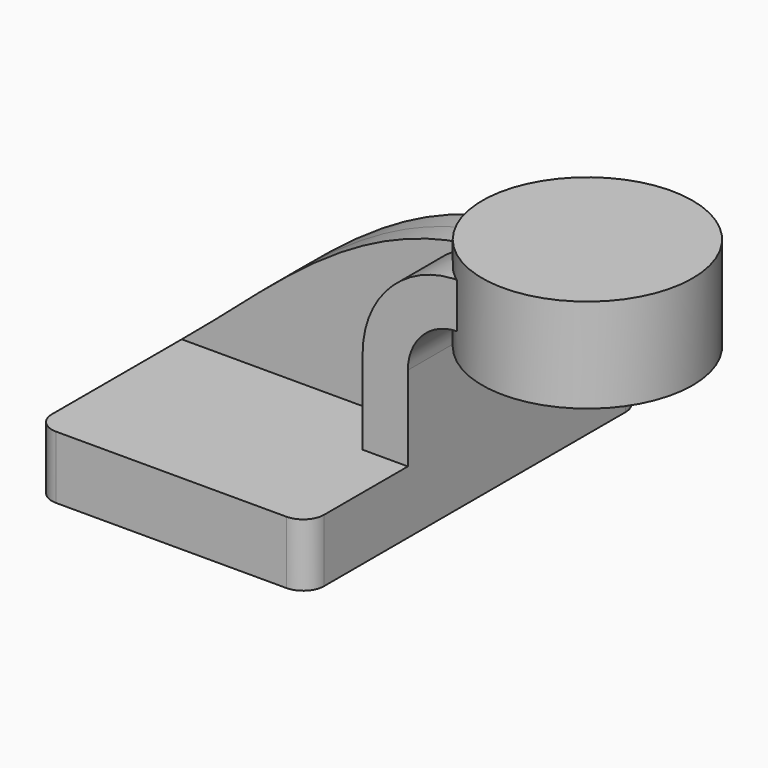
from build123d import *

# Parameters (mm, degrees)
F1_DEPTH = 63.5
F2_DEPTH = 7.9375
F3_DEPTH = 25.4
F4_R     = 6.35


# Not quite as in the source:
# - ends of sketch curves that miss each other by under 0.0002 mm in the source are joined


with BuildPart() as f1:
    # F0 (on Front) → F1 (new body, symmetric)
    with BuildSketch(Plane.XZ):
        Polygon((-41.275, 9.525), (-41.275, -9.525), (41.275, -9.525), (41.275, 9.525), (27.5589991361, 9.525), align=None)
    extrude(amount=F1_DEPTH, both=True)

    # F0 (on Front) → F2 (join, symmetric)
    with BuildSketch(Plane.XZ):
        with BuildLine():
            add(Edge.make_bspline(
                [(-41.275, 9.525), (-12.8610799571, 32.6827113613), (12.6950968294, 62.5117734864), (54.8244975817, 64.1265564996)],
                knots=[0, 0, 0, 0, 110.5540678871, 110.5540678871, 110.5540678871, 110.5540678871], degree=3))
            Line((-41.275, 9.525), (27.5589991361, 9.525))
            Line((27.5589991361, 9.525), (27.5589991361, 35.2199450135))
            ThreePointArc((27.5589991361, 35.2199450135), (35.450810299, 55.0882589398), (54.8244975817, 64.1265564996))
        make_face()
    extrude(amount=F2_DEPTH, both=True)

    # F0 (on Front) → F3 (join, symmetric)
    with BuildSketch(Plane.XZ):
        with BuildLine():
            Line((27.5589991361, 9.525), (41.275, 9.525))
            Line((41.275, 9.525), (41.275, 35.2199450135))
            ThreePointArc((41.275, 35.2199450135), (45.7386926547, 45.9962523588), (56.515, 50.4599450135))
            Line((56.515, 50.4599450135), (56.515, 64.1759467518))
            add(Edge.make_bspline(
                [(54.8244975817, 64.1265564996), (55.3850490812, 64.1480419473), (55.9485346305, 64.1645324648), (56.515, 64.1759467518)],
                knots=[110.5540678871, 110.5540678871, 110.5540678871, 110.5540678871, 112.0250417777, 112.0250417777, 112.0250417777, 112.0250417777], degree=3))
            ThreePointArc((54.8244975817, 64.1265564996), (35.450810299, 55.0882589398), (27.5589991361, 35.2199450135))
            Line((27.5589991361, 35.2199450135), (27.5589991361, 9.525))
        make_face()
    extrude(amount=F3_DEPTH, both=True)

    # F4
    f4_edges = [f1.edges().sort_by_distance(p)[0] for p in [
        (-41.275, -63.5, 0),
        (41.275, -63.5, 0),
        (41.275, 63.5, 0),
        (-41.275, 63.5, 0),
    ]]
    fillet(f4_edges, radius=F4_R)

    # F0 (on Front) → F5 (revolve)
    with BuildSketch(Plane.XZ):
        Polygon((75.4097700119, 70.9069057465), (75.4097700119, 64.1759485006), (75.4097700119, 50.4599450135), (75.4097700119, 42.3319057465), (107.315, 42.3319057465), (107.315, 70.9069057465), align=None)
    revolve(axis=Axis((75.4097700119, 0, 56.6194057465), (0, 0, 1)))


solid = f1.part
